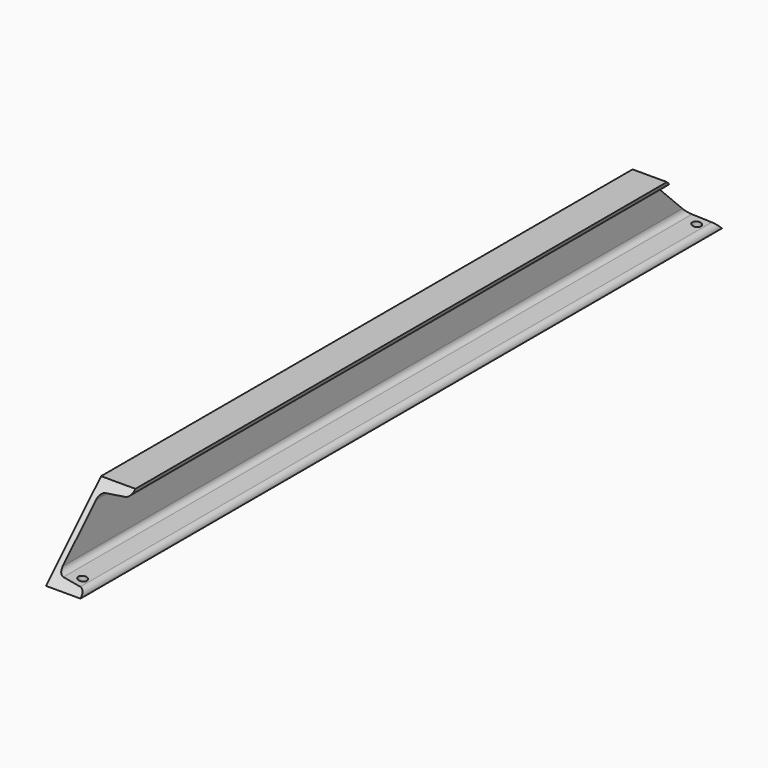
from build123d import *

# Parameters (mm, degrees)
F1_DEPTH = 444.5
F2_SIZE  = 76.19999
F3_SIZE  = 76.19999
F4_R     = 4.7625
F5_DEPTH = 25.4
F6_DEPTH = 25.4


# Not quite as in the source:
# - a fillet or chamfer is up to 0.001 mm smaller than in the source, because OpenCascade refuses the exact size


with BuildPart() as f1:
    # F0 (on Front) → F1 (new body, symmetric)
    with BuildSketch(Plane.XZ):
        with BuildLine():
            Line((34.6709999669, 34.4712352276), (-3.4290000331, 34.4712352276))
            Line((-3.4290000331, 34.4712352276), (-3.4290000331, -41.7287647724))
            Line((-3.4290000331, -41.7287647724), (34.6709999669, -41.7287647724))
            Line((34.6709999669, -41.7287647724), (34.6709999669, -41.1254357918))
            ThreePointArc((34.6709999669, -41.1254357918), (33.029223555, -36.864552005), (28.9528485827, -34.806949634))
            Line((28.9528485827, -34.806949634), (8.6391513512, -32.7755799108))
            ThreePointArc((8.6391513512, -32.7755799108), (4.5627763789, -30.7179775398), (2.9209999669, -26.457093753))
            Line((2.9209999669, -26.457093753), (2.9209999669, 19.1995642082))
            ThreePointArc((2.9209999669, 19.1995642082), (4.5627763789, 23.460447995), (8.6391513512, 25.518050366))
            Line((8.6391513512, 25.518050366), (28.9528485827, 27.5494200892))
            ThreePointArc((28.9528485827, 27.5494200892), (33.029223555, 29.6070224602), (34.6709999669, 33.867906247))
            Line((34.6709999669, 33.867906247), (34.6709999669, 34.4712352276))
        make_face()
    extrude(amount=F1_DEPTH, both=True)

    # F2 (size 76.2 in the source; OpenCascade refuses exactly that, so slightly less here)
    f2_edges = [f1.edges().sort_by_distance(p)[0] for p in [
        (15.621, -444.5, 34.471235),
    ]]
    chamfer(f2_edges, length=F2_SIZE)

    # F3 (size 76.2 in the source; OpenCascade refuses exactly that, so slightly less here)
    f3_edges = [f1.edges().sort_by_distance(p)[0] for p in [
        (15.621, 444.5, 34.471235),
    ]]
    chamfer(f3_edges, length=F3_SIZE)

    # F4 (on face) → F5 (cut)
    with BuildSketch(Plane(origin=(0, 0, -41.7287647724), x_dir=(1, 0, 0), z_dir=(0, 0, -1))):
        with Locations((21.9709999669, 425.45)):
            Circle(F4_R)
    extrude(amount=-F5_DEPTH, mode=Mode.SUBTRACT)

    # F4 (on face) → F6 (cut)
    with BuildSketch(Plane(origin=(0, 0, -41.7287647724), x_dir=(1, 0, 0), z_dir=(0, 0, -1))):
        with Locations((21.9709999669, 425.45)):
            Circle(F4_R)
        with Locations((21.9709999669, -425.45)):
            Circle(F4_R)
    extrude(amount=-F6_DEPTH, mode=Mode.SUBTRACT)


solid = f1.part
